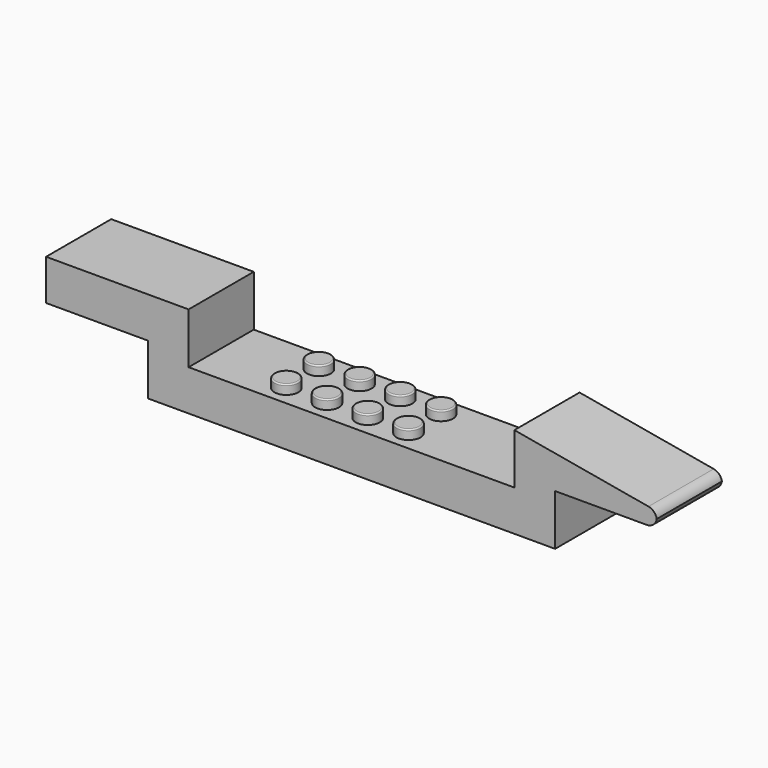
from build123d import *

# Parameters (mm, degrees)
F1_DEPTH    = 16
F2_W        = 13.0048
F2_H        = 13
F2_R        = 3.2512
F2_R_2      = 2.4003
F3_DEPTH    = 3.5
F5_R        = 2.3492063492
F6_DEPTH    = 1.85
F7_T1_DEPTH = 163.3704583371
F8_T1_DEPTH = 24.3909963118
F8_T3_DEPTH = 26
F9_R        = 0.25


# Not quite as in the source:
# - a fillet or chamfer that OpenCascade refuses, or shapes differently, is made with other operations: its cross-section is extruded or revolved along the edge and cut away or added
# - a feature names something its author has since deleted; it is built from what else it names


with BuildPart() as f1:
    # F0 (on Front) → F1 (new body)
    with BuildSketch(Plane.XZ):
        Polygon((-40, 0), (0, 0), (0, 8), (-32, 8), (-32, 18), (-60, 18), (-60, 10), (-40, 10), align=None)
    extrude(amount=-F1_DEPTH)

    # F2 (on face) → F3 (cut)
    with BuildSketch(Plane(origin=(0, 0, 10), x_dir=(1, 0, 0), z_dir=(0, 0, -1))):
        with Locations((-50, -8)):
            Rectangle(F2_W, F2_H)
        with Locations((-50, -8)):
            Circle(F2_R, mode=Mode.SUBTRACT)
        with Locations((-50, -8)):
            Circle(F2_R_2)
    extrude(amount=-F3_DEPTH, mode=Mode.SUBTRACT)

    # F4: F1 across face


with BuildPart() as f1_1:
    add(f1.part)
    add(f1.part.mirror(Plane(origin=(0, 8, 4), x_dir=(0, 1, 0), z_dir=(1, 0, 0))))

    # F5 (on face) → F6 (join)
    with BuildSketch(Plane.XY.offset(8)):
        with Locations((-16, 4)):
            Circle(F5_R)
        with Locations((-16, 12)):
            Circle(F5_R)
        with Locations((-8, 12)):
            Circle(F5_R)
        with Locations((-8, 4)):
            Circle(F5_R)
        with Locations((0, 4)):
            Circle(F5_R)
        with Locations((0, 12)):
            Circle(F5_R)
        with Locations((8, 12)):
            Circle(F5_R)
        with Locations((8, 4)):
            Circle(F5_R)
    extrude(amount=F6_DEPTH)

    # F7: chamfer of 5 x 28.3564090981 on 1 edges, made by hand

    # F7_s2 → F7_t1 (cut)
    with BuildSketch(Plane.XZ.offset(-89.6852291686)):
        Polygon((60, 13), (31.6435909019, 18), (60, 18), align=None)
    extrude(amount=F7_T1_DEPTH, mode=Mode.SUBTRACT)

    # F8: fillet of radius 2 on 2 edges, made by hand

    # F8_s2 → F8_t1 (cut)
    with BuildSketch(Plane.XZ.offset(-20.1954981559)):
        with BuildLine():
            ThreePointArc((58.3472963553, 13.2914162437), (59.5320888862, 12.607375957), (60, 11.3218007376))
            Line((60, 11.3218007376), (60, 13))
            Line((60, 13), (58.3472963553, 13.2914162437))
        make_face()
    extrude(amount=F8_T1_DEPTH, mode=Mode.SUBTRACT)

    # F8_s4 → F8_t3 (cut)
    with BuildSketch(Plane.XZ.offset(-21)):
        with BuildLine():
            ThreePointArc((60, 12), (59.4142135624, 10.5857864376), (58, 10))
            Line((58, 10), (60, 10))
            Line((60, 10), (60, 12))
        make_face()
    extrude(amount=F8_T3_DEPTH, mode=Mode.SUBTRACT)

    # F9
    f9_edges = [f1_1.edges().sort_by_distance(p)[0] for p in [
        (-18.349206, 4, 9.85),
        (-18.349206, 12, 9.85),
        (-10.349206, 12, 9.85),
        (-10.349206, 4, 9.85),
        (-2.349206, 4, 9.85),
        (-2.349206, 12, 9.85),
        (5.650794, 12, 9.85),
        (5.650794, 4, 9.85),
    ]]
    fillet(f9_edges, radius=F9_R)


solid = f1_1.part
